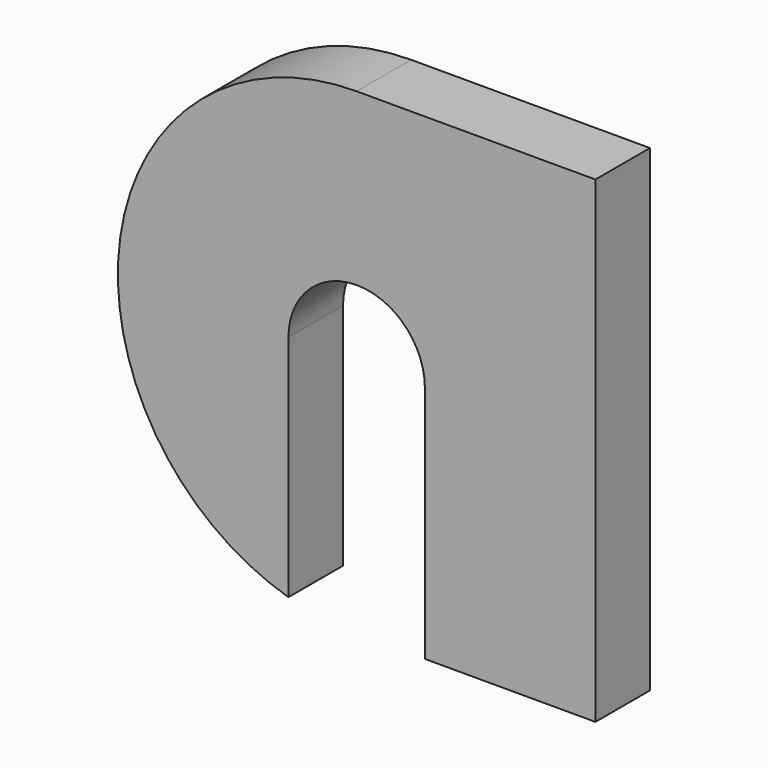
from build123d import *

# Parameters (mm, degrees)
F2_DEPTH = 6.35


# Not quite as in the source:
# - a feature of the source that left no trace in its solid (it failed there, or was rolled back) is left out
# - a feature names something its author has since deleted; it is built from what else it names


with BuildPart() as f2:
    # F0 (on Front) → F2 (new body)
    with BuildSketch(Plane.XZ):
        with BuildLine():
            Line((6.35, -22.225), (22.225, -22.225))
            Line((22.225, -22.225), (22.225, 22.225))
            Line((22.225, 22.225), (0, 22.225))
            ThreePointArc((0, 22.225), (-15.7154482119, 15.7154482119), (-22.225, 0))
            ThreePointArc((-22.225, 0), (-17.8196433045, -13.2819779212), (-6.35, -21.2985474857))
            Line((-6.35, -21.2985474857), (-6.35, 0))
            ThreePointArc((-6.35, 0), (0, 6.35), (6.35, 0))
            Line((6.35, 0), (6.35, -22.225))
        make_face()
    extrude(amount=F2_DEPTH)


with BuildPart() as f2_1:
    # F3: moved
    add(f2.part.moved(Location((-22.225, -50.8, 0))))


solid = f2_1.part
